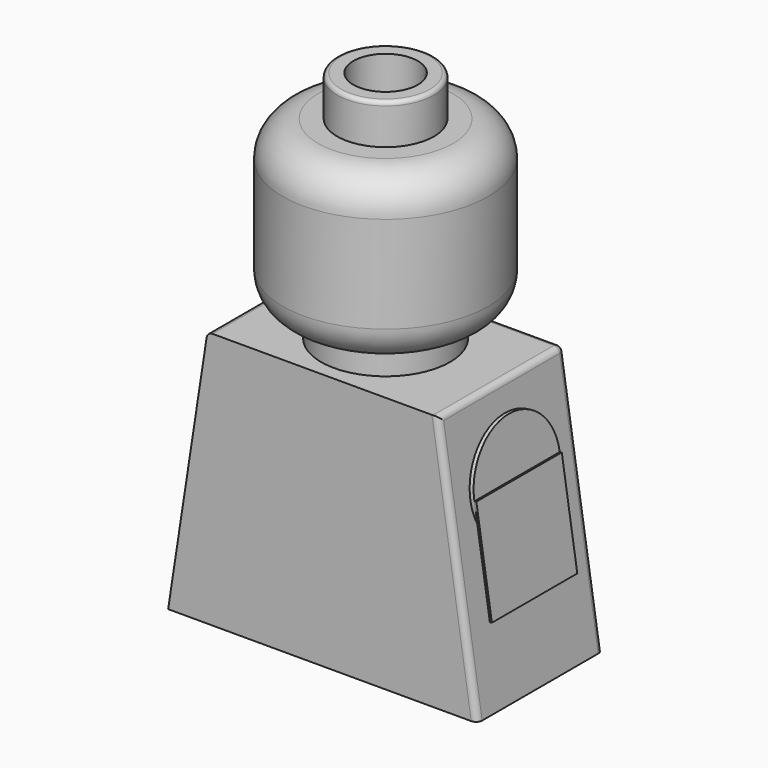
from build123d import *
from build123d import SkipClean  # not in build123d's __all__

# Parameters (mm, degrees)
F3_DEPTH  = 25
F4_R      = 2.4
F5_DEPTH  = 5.8
F7_DEPTH  = 3.9
F8_T      = -1.35
F10_DEPTH = 11.4
F12_R     = 2
F13_DEPTH = 1.35
F11_R     = 2
F14_DEPTH = 1.35
F15_R     = 0.3
F16_R     = 2.65
F16_R_2   = 2
F17_DEPTH = 0.2
F19_DEPTH = 0.1


with BuildPart() as f1:
    # F0 (on Front) → F1 (revolve)
    with BuildSketch(Plane.XZ):
        with BuildLine():
            Line((2.5, 0), (3.2, 0))
            Line((3.2, 0), (3.2, 1.3))
            Line((3.2, 1.3), (3.35, 1.3))
            ThreePointArc((3.35, 1.3), (4.5874368671, 1.8125631329), (5.1, 3.05))
            Line((5.1, 3.05), (5.1, 7.85))
            ThreePointArc((5.1, 7.85), (4.5874368671, 9.0874368671), (3.35, 9.6))
            Line((3.35, 9.6), (2.4, 9.6))
            Line((2.4, 9.6), (2.4, 11.4))
            ThreePointArc((2.4, 11.4), (2.3414213562, 11.5414213562), (2.2, 11.6))
            Line((2.2, 11.6), (1.6, 11.6))
            Line((1.6, 11.6), (1.6, 9.6))
            Line((1.6, 9.6), (0, 9.6))
            Line((0, 9.6), (0, 8.6))
            Line((0, 8.6), (2.5, 8.6))
            Line((2.5, 8.6), (2.5, 0))
        make_face()
    revolve(axis=Axis((0, 0, 5.8), (0, 0, 1)))

    # F2 (on face) → F3 (cut)
    with BuildSketch(Plane.XY.offset(9.6)):
        with BuildLine():
            Line((-1.5491933385, 0.4), (-0.2309401077, 0.4))
            Line((-0.2309401077, 0.4), (0.4281865077, 1.5416407865))
            ThreePointArc((0.4281865077, 1.5416407865), (-0.8, 1.3856406461), (-1.5491933385, 0.4))
        make_face()
        with BuildLine():
            Line((1.1210068308, 1.1416407865), (0.4618802154, 0))
            Line((0.4618802154, 0), (1.1210068308, -1.1416407865))
            ThreePointArc((1.1210068308, -1.1416407865), (1.4754001032, -0.6190270878), (1.6, 0))
            ThreePointArc((1.6, 0), (1.4754001032, 0.6190270878), (1.1210068308, 1.1416407865))
        make_face()
        with BuildLine():
            Line((0.4281865077, -1.5416407865), (-0.2309401077, -0.4))
            Line((-0.2309401077, -0.4), (-1.5491933385, -0.4))
            ThreePointArc((-1.5491933385, -0.4), (-0.8, -1.3856406461), (0.4281865077, -1.5416407865))
        make_face()
    with SkipClean():  # cleaning this boolean's faces spoils the solid; the shape is the same uncleaned
        extrude(amount=-F3_DEPTH, mode=Mode.SUBTRACT)


with BuildPart() as f5:
    # F4 (on face) → F5 (new body)
    with BuildSketch(Plane(origin=(0, 0, 0), x_dir=(1, 0, 0), z_dir=(0, 0, -1))):
        Circle(F4_R)
    extrude(amount=-F5_DEPTH)

    # F6 (on Front) → F7 (join, symmetric)
    with BuildSketch(Plane.XZ):
        Polygon((5.725, 0), (-5.725, 0), (-7.675, -12.75), (7.675, -12.75), align=None)
    extrude(amount=F7_DEPTH, both=True)

    # F8
    f8_openings = [f5.faces().sort_by_distance(p)[0] for p in [
        (0, 0, -12.75),
    ]]
    offset(amount=F8_T, openings=f8_openings, kind=Kind.INTERSECTION)

    # F9 (on face) → F10 (join, through all)
    with BuildSketch(Plane(origin=(0, 0, -1.35), x_dir=(1, 0, 0), z_dir=(0, 0, -1))):
        Polygon((-1.856, 1.95), (-1.856, 2.55), (-2.456, 2.55), align=None)
        Polygon((2.456, 2.55), (1.856, 2.55), (1.856, 1.95), align=None)
        Polygon((-1.856, -1.95), (-2.456, -2.55), (-1.856, -2.55), align=None)
        Polygon((1.856, -2.55), (2.456, -2.55), (1.856, -1.95), align=None)
    extrude(amount=F10_DEPTH)

    # F12 (on face) → F13 (cut)
    with BuildSketch(Plane(origin=(-5.5941472816, 0, 0.8555754666), x_dir=(0, -1, 0), z_dir=(-0.9885057562, 0, 0.1511832333))):
        with Locations((0, -4.8655240106)):
            Circle(F12_R)
    extrude(amount=-F13_DEPTH, mode=Mode.SUBTRACT)

    # F11 (on face) → F14 (cut)
    with BuildSketch(Plane(origin=(5.5941472816, 0, 0.8555754666), x_dir=(0, 1, 0), z_dir=(0.9885057562, 0, 0.1511832333))):
        with Locations((0, -4.8655240106)):
            Circle(F11_R)
    extrude(amount=-F14_DEPTH, mode=Mode.SUBTRACT)

    # F15
    f15_edges = [f5.edges().sort_by_distance(p)[0] for p in [
        (-6.7, 3.9, -6.375),
        (0, 3.9, 0),
        (-5.725, 0, 0),
        (6.7, 3.9, -6.375),
        (5.725, 0, 0),
        (6.7, -3.9, -6.375),
    ]]
    fillet(f15_edges, radius=F15_R)


with BuildPart() as f17:
    # F16 (on face) → F17 (new body)
    with BuildSketch(Plane(origin=(5.5941472816, 0, 0.8555754666), x_dir=(0, 1, 0), z_dir=(0.9885057562, 0, 0.1511832333))):
        with Locations((0, -4.8655240106)):
            Circle(F16_R)
        with Locations((0, -4.8655240106)):
            Circle(F16_R_2, mode=Mode.SUBTRACT)
        with Locations((0, -4.8655240106)):
            Circle(F16_R_2)
    extrude(amount=F17_DEPTH)

    # F18 (on face) → F19 (join)
    with BuildSketch(Plane(origin=(5.7918484328, 0, 0.8858121133), x_dir=(0, 1, 0), z_dir=(0.9885057562, 0, 0.1511832333))):
        with BuildLine():
            Line((2.65, -9.9655240106), (2.65, -4.8655240106))
            ThreePointArc((2.65, -4.8655240106), (0, -7.5155240106), (-2.65, -4.8655240106))
            Line((-2.65, -4.8655240106), (-2.65, -9.9655240106))
            Line((-2.65, -9.9655240106), (2.65, -9.9655240106))
        make_face()
        with BuildLine():
            ThreePointArc((-2.65, -4.8655240106), (0, -7.5155240106), (2.65, -4.8655240106))
            Line((2.65, -4.8655240106), (0, -4.8655240106))
            Line((0, -4.8655240106), (-2.65, -4.8655240106))
        make_face()
    extrude(amount=F19_DEPTH)


solid = Compound([f1.part, f5.part, f17.part])
